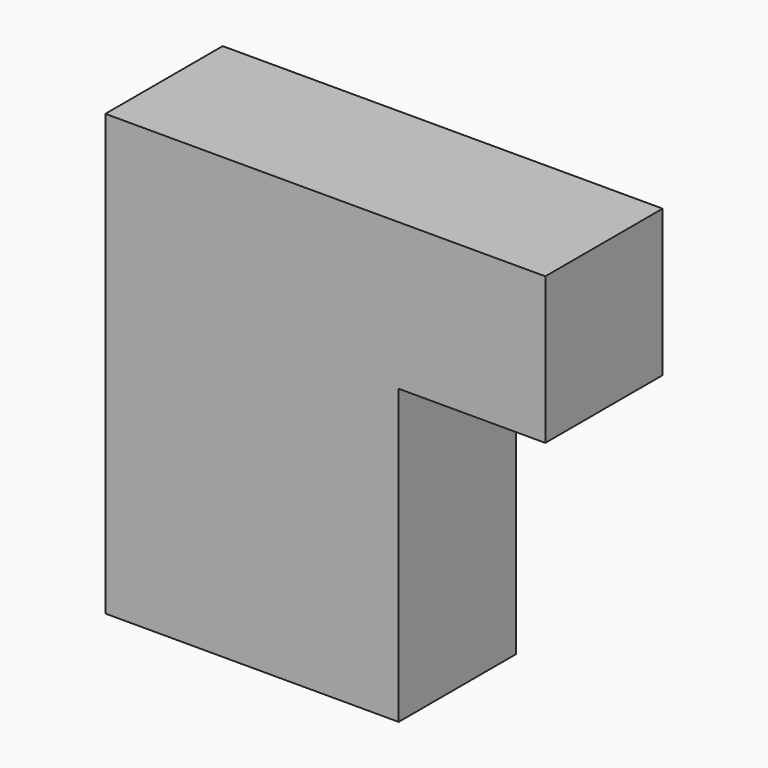
from build123d import *

# Parameters (mm, degrees)
F1_W     = 228.6
F1_H     = 228.6
F2_DEPTH = 76.2
F3_W     = 76.2
F3_H     = 152.4
F4_DEPTH = 76.201


# Not quite as in the source:
# - a variable given as a bare number and used for a length is read in inches; the dataset says mm whatever the document's units were


with BuildPart() as f2:
    # F1 (on Front) → F2 (new body)
    with BuildSketch(Plane.XZ):
        Rectangle(F1_W, F1_H)
    extrude(amount=F2_DEPTH)

    # F3 (on face) → F4 (cut, through all)
    with BuildSketch(Plane.XZ.offset(76.2)):
        with Locations((76.2, -38.1)):
            Rectangle(F3_W, F3_H)
    extrude(amount=-F4_DEPTH, mode=Mode.SUBTRACT)


solid = f2.part
